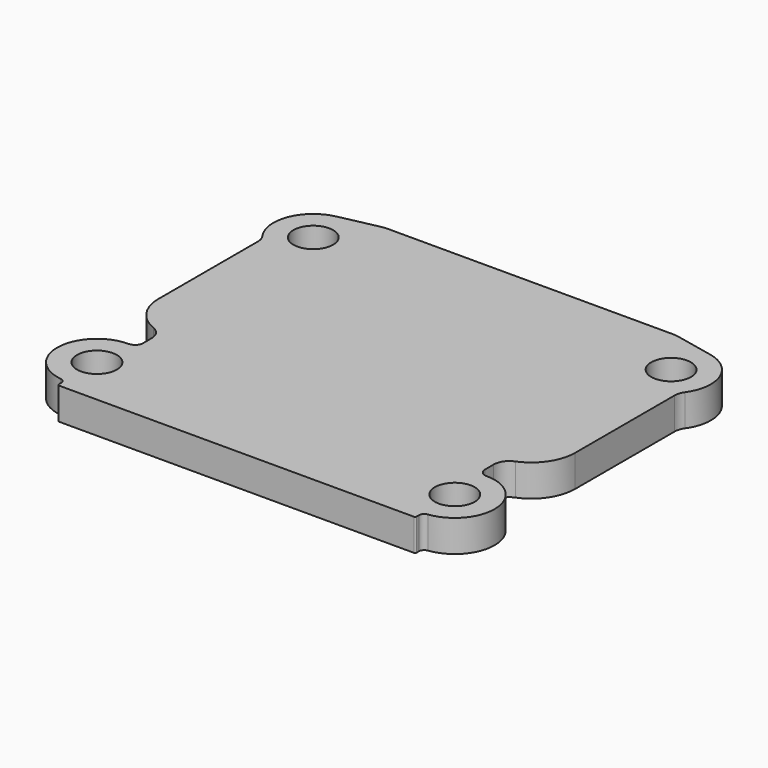
from build123d import *

# Parameters (mm, degrees)
F0_R     = 2.5
F1_DEPTH = 4
F2_R     = 2
F3_R     = 1
F4_R     = 0.7
F5_R     = 0.2
F6_R     = 2
F7_R     = 5


with BuildPart() as f1:
    # F0 (on Top) → F1 (new body)
    with BuildSketch(Plane.XY):
        with BuildLine():
            Line((-44, 8.8584928558), (-44, 4.8989794856))
            ThreePointArc((-44, 4.8989794856), (-49.974680765, 0.50254481), (-45, -5))
            Line((-45, -5), (-45, -6.2))
            Line((-45, -6.2), (0, -6.2))
            Line((0, -6.2), (0, -5))
            ThreePointArc((0, -5), (4.974680765, 0.50254481), (-1, 4.8989794856))
            Line((-1, 4.8989794856), (-1, 8.8584928558))
            ThreePointArc((-1, 8.8584928558), (2.3623310777, 10.7048643976), (3.7, 14.3))
            Line((3.7, 14.3), (3.7, 30.6369656558))
            ThreePointArc((3.7, 30.6369656558), (4.7588909504, 35.5339351103), (1.0395584541, 38.8907380037))
            Line((1.0395584541, 38.8907380037), (-4.1791089332, 40))
            Line((-4.1791089332, 40), (-40.8208910668, 40))
            Line((-40.8208910668, 40), (-46.0395584541, 38.8907380037))
            ThreePointArc((-46.0395584541, 38.8907380037), (-49.7588909504, 35.5339351103), (-48.7, 30.6369656558))
            Line((-48.7, 30.6369656558), (-48.7, 14.3))
            ThreePointArc((-48.7, 14.3), (-47.3623310777, 10.7048643976), (-44, 8.8584928558))
        make_face()
        with Locations((-45, 0)):
            Circle(F0_R, mode=Mode.SUBTRACT)
        Circle(F0_R, mode=Mode.SUBTRACT)
        with Locations((-45, 34)):
            Circle(F0_R, mode=Mode.SUBTRACT)
        with Locations((0, 34)):
            Circle(F0_R, mode=Mode.SUBTRACT)
    extrude(amount=F1_DEPTH)

    # F2
    f2_edges = [f1.edges().sort_by_distance(p)[0] for p in [
        (-44, 8.858493, 2),
        (-1, 8.858493, 2),
    ]]
    fillet(f2_edges, radius=F2_R)

    # F3
    f3_edges = [f1.edges().sort_by_distance(p)[0] for p in [
        (-1, 4.898979, 2),
        (-44, 4.898979, 2),
    ]]
    fillet(f3_edges, radius=F3_R)

    # F4
    f4_edges = [f1.edges().sort_by_distance(p)[0] for p in [
        (-45, -5, 2),
        (0, -5, 2),
    ]]
    fillet(f4_edges, radius=F4_R)

    # F5
    f5_edges = [f1.edges().sort_by_distance(p)[0] for p in [
        (-45, -6.2, 2),
        (0, -6.2, 2),
    ]]
    fillet(f5_edges, radius=F5_R)

    # F6
    f6_edges = [f1.edges().sort_by_distance(p)[0] for p in [
        (-48.7, 30.636966, 2),
        (3.7, 30.636966, 2),
    ]]
    fillet(f6_edges, radius=F6_R)

    # F7
    f7_edges = [f1.edges().sort_by_distance(p)[0] for p in [
        (-40.820891, 40, 2),
        (-4.179109, 40, 2),
    ]]
    fillet(f7_edges, radius=F7_R)


solid = f1.part
